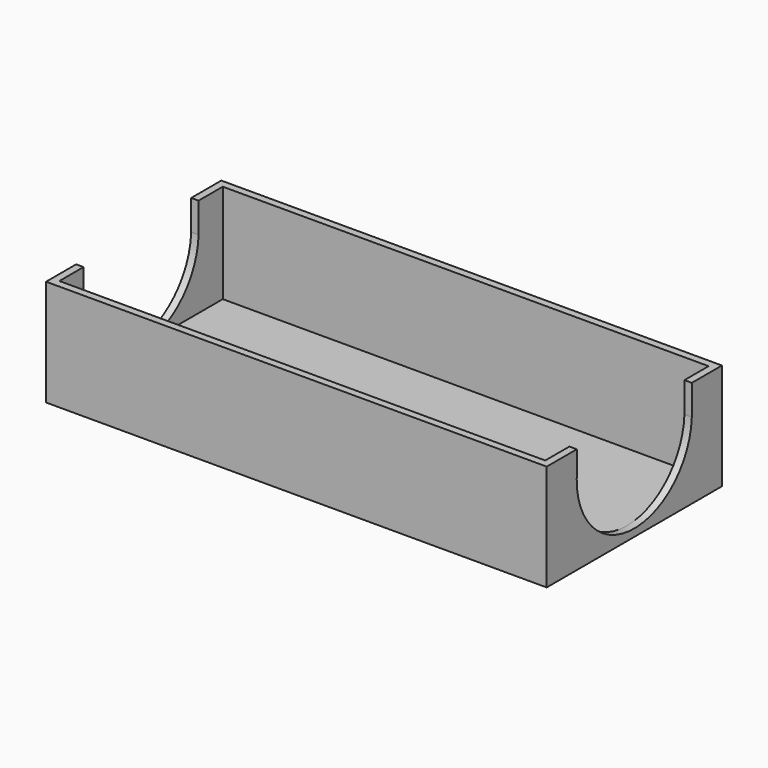
from build123d import *

# Parameters (mm, degrees)
F0_W     = 101.6
F0_H     = 44.45
F1_DEPTH = 21.59
F2_T     = -1.5
F4_DEPTH = 1.5


# Not quite as in the source:
# - a pattern or mirror of a feature is missing from the dataset's text; its kind, count and spacing are read off the source's solid


with BuildPart() as f1:
    # F0 (on Top) → F1 (new body)
    with BuildSketch(Plane.XY):
        Rectangle(F0_W, F0_H)
    extrude(amount=F1_DEPTH)

    # F2
    f2_openings = [f1.faces().sort_by_distance(p)[0] for p in [
        (0, 0, 21.59),
    ]]
    offset(amount=F2_T, openings=f2_openings)

    # F3 (on face) → F4 (cut)
    with BuildSketch(Plane(origin=(-50.8, 0, 0), x_dir=(0, -1, 0), z_dir=(-1, 0, 0))):
        with BuildLine():
            ThreePointArc((-14.5911212754, 15.4684429111), (0.3183541842, 1.5034700934), (14.605, 16.105))
            ThreePointArc((14.605, 16.105), (14.6032460444, 16.3313403807), (14.5979845987, 16.5576263976))
            ThreePointArc((14.5979845987, 16.5576263976), (14.290212434, 19.1209332868), (13.5359078011, 21.59))
            Line((13.5359078011, 21.59), (-13.5359078011, 21.59))
            ThreePointArc((-13.5359078011, 21.59), (-14.2709246664, 19.2109192145), (-14.5911212754, 16.7415570889))
            Line((-14.5911212754, 16.7415570889), (-14.5911212754, 15.4684429111))
        make_face()
        with BuildLine():
            ThreePointArc((13.5359078011, 21.59), (14.290212434, 19.1209332868), (14.5979845987, 16.5576263976))
            Line((14.5979845987, 16.5576263976), (14.5979845987, 21.59))
            Line((14.5979845987, 21.59), (13.5359078011, 21.59))
        make_face()
        with BuildLine():
            Line((-14.5911212754, 21.59), (-14.5911212754, 16.7415570889))
            ThreePointArc((-14.5911212754, 16.7415570889), (-14.2709246664, 19.2109192145), (-13.5359078011, 21.59))
            Line((-13.5359078011, 21.59), (-14.5911212754, 21.59))
        make_face()
    f4 = extrude(amount=-F4_DEPTH, mode=Mode.SUBTRACT)

    # F4_copies: F4 across plane
    add(f4.mirror(Plane(origin=(0, 0, 0), x_dir=(0, 0, 1), z_dir=(1, 0, 0))), mode=Mode.SUBTRACT)


solid = f1.part
